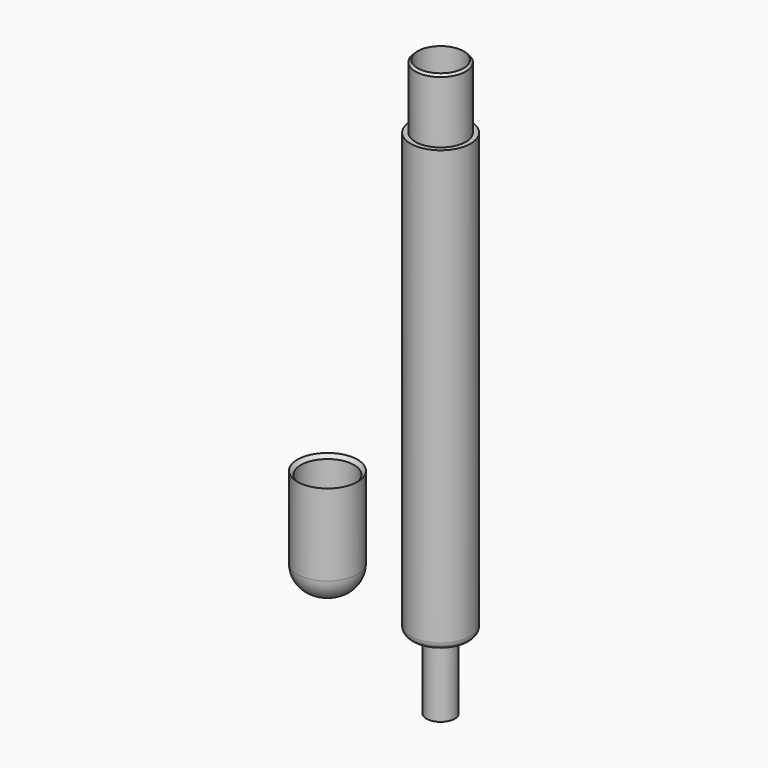
from build123d import *

# Parameters (mm, degrees)
F0_R     = 6.5
F0_R_2   = 4
F1_DEPTH = 3
F0_R_3   = 7.5
F2_DEPTH = 10
F0_R_4   = 8.5
F3_DEPTH = 30
F0_R_5   = 7.125
F4_DEPTH = 143
F5_DEPTH = 124.5
F6_R     = 7
F7_R     = 2
F9_DEPTH = 20


# Not quite as in the source:
# - a fillet or chamfer that OpenCascade refuses, or shapes differently, is made with other operations: its cross-section is extruded or revolved along the edge and cut away or added


with BuildPart() as f1:
    # F0 (on Top) → F1 (new body)
    with BuildSketch(Plane.XY):
        Circle(F0_R)
        Circle(F0_R_2, mode=Mode.SUBTRACT)
        Circle(F0_R_2)
    extrude(amount=F1_DEPTH)

    # F0 (on Top) → F4 (join)
    with BuildSketch(Plane.XY):
        Circle(F0_R_5)
        Circle(F0_R, mode=Mode.SUBTRACT)
    extrude(amount=F4_DEPTH)

    # F0 (on Top) → F5 (join)
    with BuildSketch(Plane.XY):
        Circle(F0_R_4)
        Circle(F0_R_5, mode=Mode.SUBTRACT)
    extrude(amount=F5_DEPTH)

    # F7
    f7_edges = [f1.edges().sort_by_distance(p)[0] for p in [
        (-8.5, 0, 0),
    ]]
    fillet(f7_edges, radius=F7_R)

    # F8: chamfer of 1 on 1 edges, made by hand

    # F8_s1 → F8_t2 (revolve, cut)
    with BuildSketch(Plane.XZ):
        Polygon((7.125, 142), (6.125, 143), (7.125, 143), align=None)
    revolve(axis=Axis((0, 0, 143), (0, 0, 1)), mode=Mode.SUBTRACT)

    # F0 (on Top) → F9 (join)
    with BuildSketch(Plane.XY):
        Circle(F0_R_2)
    extrude(amount=-F9_DEPTH)


with BuildPart() as f1b:
    # F0 (on Top) → F1, piece 2 (new body)
    with BuildSketch(Plane.XY):
        with Locations((-31.9685041904, 0)):
            Circle(F0_R)
    extrude(amount=F1_DEPTH)

    # F0 (on Top) → F2 (join)
    with BuildSketch(Plane.XY):
        with Locations((-31.9685041904, 0)):
            Circle(F0_R_3)
        with Locations((-31.9685041904, 0)):
            Circle(F0_R, mode=Mode.SUBTRACT)
    extrude(amount=F2_DEPTH)

    # F0 (on Top) → F3 (join)
    with BuildSketch(Plane.XY):
        with Locations((-31.9685041904, 0)):
            Circle(F0_R_4)
        with Locations((-31.9685041904, 0)):
            Circle(F0_R_3, mode=Mode.SUBTRACT)
    extrude(amount=F3_DEPTH)

    # F6
    f6_edges = [f1b.edges().sort_by_distance(p)[0] for p in [
        (-40.468504, 0, 0),
    ]]
    fillet(f6_edges, radius=F6_R)

    # F8#2: chamfer of 1 on 1 edges, made by hand

    # F8_2_s1 → F8_2_t2 (revolve, cut)
    with BuildSketch(Plane.XZ):
        Polygon((-23.4685041904, 30), (-24.4685041904, 29), (-24.4685041904, 30), align=None)
    revolve(axis=Axis((-31.9685041904, 0, 30), (0, 0, 1)), mode=Mode.SUBTRACT)


solid = Compound([f1.part, f1b.part])
